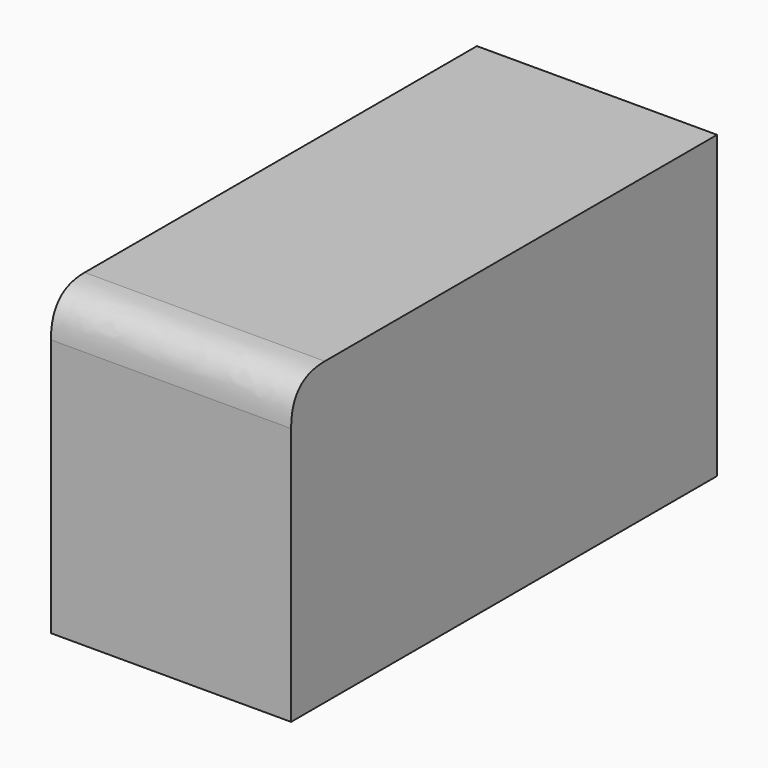
from build123d import *

# Parameters (mm, degrees)
F0_W        = 160.4959368706
F0_H        = 90.5437916517
F1_DEPTH    = 72.39
F2_T1_DEPTH = 135.89


# Not quite as in the source:
# - a fillet or chamfer that OpenCascade refuses, or shapes differently, is made with other operations: its cross-section is extruded or revolved along the edge and cut away or added


with BuildPart() as f1:
    # F0 (on Right) → F1 (new body)
    with BuildSketch(Plane.YZ):
        Rectangle(F0_W, F0_H)
    extrude(amount=F1_DEPTH)

    # F2: fillet of radius 12.7 on 1 edges, made by hand

    # F2_s2 → F2_t1 (cut)
    with BuildSketch(Plane.YZ.offset(-31.75)):
        with BuildLine():
            add(Edge.make_bspline(
                [(-67.5479684353, 45.2718958259), (-80.2479684353, 45.2718958259), (-80.2479684353, 32.5718958259)],
                knots=[0, 0, 0, 1, 1, 1], degree=2, weights=[1, 1, 1]))
            Line((-80.2479684353, 32.5718958259), (-80.2479684353, 45.2718958259))
            Line((-80.2479684353, 45.2718958259), (-67.5479684353, 45.2718958259))
        make_face()
    extrude(amount=F2_T1_DEPTH, mode=Mode.SUBTRACT)


solid = f1.part
